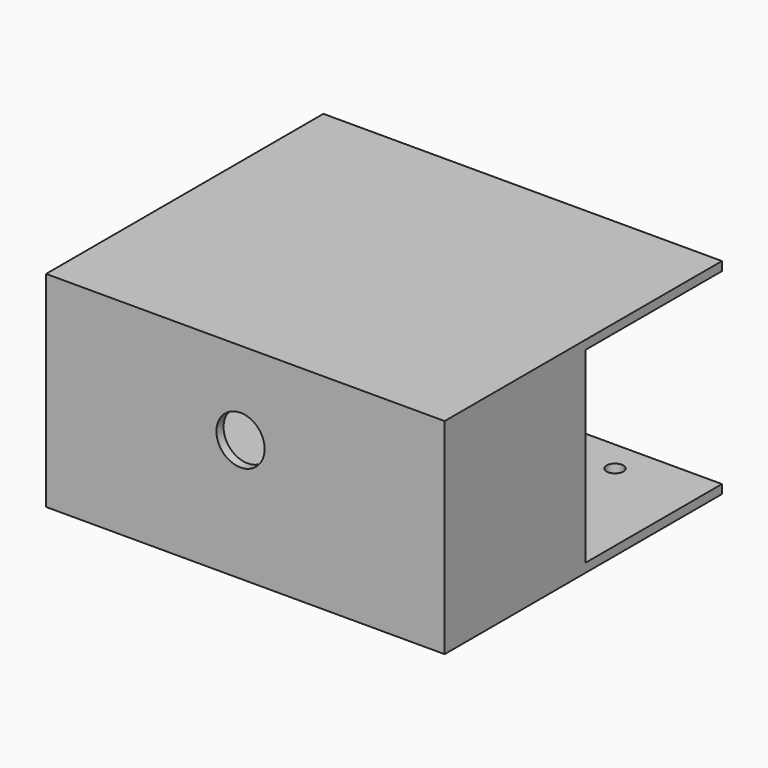
from build123d import *
from build123d import SkipClean  # not in build123d's __all__

# Parameters (mm, degrees)
F0_W             = 57.5
F0_H             = 50
F1_DEPTH         = 107.5
F2_W             = 55.8
F2_H             = 19
F3_DEPTH         = 42
F4_W             = 0.3
F4_H             = 19
F5_DEPTH         = 48.3
F6_T1_DEPTH      = 65.5
F6_T3_DEPTH      = 67.5
F6_T5_DEPTH      = 225
F6_T7_DEPTH      = 11.7
F6_T9_DEPTH      = 11.7
F6_T11_DEPTH     = 204
F8_W             = 87
F8_H             = 15.3
F9_DEPTH         = 14
F10_W            = 8.2
F10_H            = 14
F11_DEPTH        = 7.4
F12_R            = 2
F13_R            = 2.5
F14_DEPTH        = 4
F15_R            = 1
F19_D            = 3.3
F19_DEPTH        = 5
F19_TIP          = 0.9914200214
F19_ON_F18_D     = 3.3
F19_ON_F18_DEPTH = 5
F19_ON_F18_TIP   = 0.9914200214
F19_ON_F17_D     = 3.3
F19_ON_F17_DEPTH = 5
F19_ON_F17_TIP   = 0.9914200214
F20_W            = 264
F20_H            = 50
F20_R            = 1.5
F21_DEPTH        = 6
F22_W            = 122
F22_H            = 91
F22_R            = 2.25
F23_DEPTH        = 2.4
F24_W            = 91
F24_H            = 52.9
F24_R            = 1.75
F25_DEPTH        = 2.4
F26_R            = 2.25
F27_DEPTH        = 25
F28_W            = 91
F28_H            = 52.9
F29_DEPTH        = 3
F30_R            = 1.75
F31_DEPTH        = 25
F32_W            = 127.4
F32_H            = 91
F33_DEPTH        = 2.4
F34_W            = 127.4
F34_H            = 55.3
F34_R            = 6.5
F35_DEPTH        = 2.4
F36_W            = 21.5
F36_H            = 28.5
F37_DEPTH        = 25
F38_W            = 20
F38_H            = 100
F39_DEPTH        = 60
F43_W            = 2.4
F43_H            = 50.5
F44_DEPTH        = 45


# Not quite as in the source:
# - a fillet or chamfer that OpenCascade refuses, or shapes differently, is made with other operations: its cross-section is extruded or revolved along the edge and cut away or added


with BuildPart() as f1:
    # F0 (on Front) → F1 (new body, symmetric)
    with BuildSketch(Plane.XZ):
        with Locations((-28.75, 0)):
            Rectangle(F0_W, F0_H)
    extrude(amount=F1_DEPTH, both=True)

    # F2 (on face) → F3 (cut)
    with BuildSketch(Plane.XY.offset(25)):
        with Locations((-27.9, -98)):
            Rectangle(F2_W, F2_H)
    extrude(amount=-F3_DEPTH, mode=Mode.SUBTRACT)

    # F4 (on face) → F5 (cut)
    with BuildSketch(Plane.XY.offset(25)):
        Polygon((-55.8, 107.5), (-55.8, -88.5), (-55.5, -88.5), (-55.5, 105.5), (0, 105.5), (0, 105.8), (-55.5, 105.8), (-55.5, 107.5), align=None)
        with Locations((-55.65, -98)):
            Rectangle(F4_W, F4_H)
    extrude(amount=-F5_DEPTH, mode=Mode.SUBTRACT)

    # F6: fillet of radius 2 on 9 edges, made by hand

    # F6_s2 → F6_t1 (cut)
    with BuildSketch(Plane.YZ.offset(-60.5)):
        with BuildLine():
            ThreePointArc((-86.5, 25), (-87.9142135624, 24.4142135624), (-88.5, 23))
            Line((-88.5, 23), (-88.5, 25))
            Line((-88.5, 25), (-86.5, 25))
        make_face()
        with BuildLine():
            ThreePointArc((103.5, 25), (104.9142135624, 24.4142135624), (105.5, 23))
            Line((105.5, 23), (105.5, 25))
            Line((105.5, 25), (103.5, 25))
        make_face()
    extrude(amount=F6_T1_DEPTH, mode=Mode.SUBTRACT)

    # F6_s4 → F6_t3 (cut)
    with BuildSketch(Plane.YZ.offset(-62.5)):
        with BuildLine():
            ThreePointArc((-105.5, -25), (-106.9142135624, -24.4142135624), (-107.5, -23))
            Line((-107.5, -23), (-107.5, -25))
            Line((-107.5, -25), (-105.5, -25))
        make_face()
        with BuildLine():
            ThreePointArc((105.5, -25), (106.9142135624, -24.4142135624), (107.5, -23))
            Line((107.5, -23), (107.5, -25))
            Line((107.5, -25), (105.5, -25))
        make_face()
    extrude(amount=F6_T3_DEPTH, mode=Mode.SUBTRACT)

    # F6_s6 → F6_t5 (cut)
    with BuildSketch(Plane.XZ.offset(-112.5)):
        with BuildLine():
            ThreePointArc((-55.5, -25), (-56.9142135624, -24.4142135624), (-57.5, -23))
            Line((-57.5, -23), (-57.5, -25))
            Line((-57.5, -25), (-55.5, -25))
        make_face()
    extrude(amount=F6_T5_DEPTH, mode=Mode.SUBTRACT)

    # F6_s8 → F6_t7 (cut)
    with BuildSketch(Plane.YZ.offset(-62.5)):
        with BuildLine():
            ThreePointArc((-105.5, 25), (-106.9142135624, 24.4142135624), (-107.5, 23))
            Line((-107.5, 23), (-107.5, 25))
            Line((-107.5, 25), (-105.5, 25))
        make_face()
        with BuildLine():
            ThreePointArc((105.5, 25), (106.9142135624, 24.4142135624), (107.5, 23))
            Line((107.5, 23), (107.5, 25))
            Line((107.5, 25), (105.5, 25))
        make_face()
    extrude(amount=F6_T7_DEPTH, mode=Mode.SUBTRACT)

    # F6_s10 → F6_t9 (cut)
    with BuildSketch(Plane.XZ.offset(-112.5)):
        with BuildLine():
            ThreePointArc((-55.5, 23), (-54.9142135624, 24.4142135624), (-53.5, 25))
            Line((-53.5, 25), (-55.5, 25))
            Line((-55.5, 25), (-55.5, 23))
        make_face()
    extrude(amount=F6_T9_DEPTH, mode=Mode.SUBTRACT)

    # F6_s12 → F6_t11 (cut)
    with BuildSketch(Plane.XZ.offset(-110.5)):
        with BuildLine():
            ThreePointArc((-53.5, 25), (-54.9142135624, 24.4142135624), (-55.5, 23))
            Line((-55.5, 23), (-55.5, 25))
            Line((-55.5, 25), (-53.5, 25))
        make_face()
    with SkipClean():  # cleaning this boolean's faces spoils the solid; the shape is the same uncleaned
        extrude(amount=F6_T11_DEPTH, mode=Mode.SUBTRACT)

    # F7: F1 across plane


with BuildPart() as f1_1:
    add(f1.part, clean=False)
    add(f1.part.mirror(Plane.YZ), clean=False)

    # F19
    with Locations(Plane(origin=(-57.5, 0, 0), x_dir=(0, -1, 0), z_dir=(-1, 0, 0))):
        with Locations((-75, -13), (75, -13)):
            Hole(F19_D / 2, depth=F19_DEPTH)
            with Locations((0, 0, -(F19_DEPTH + F19_TIP / 2))):  # 118° drill point
                Cone(0, F19_D / 2, F19_TIP, mode=Mode.SUBTRACT)

    # F19 on F18
    with Locations(Plane(origin=(0, 0, -25), x_dir=(1, 0, 0), z_dir=(0, 0, -1))):
        with Locations((-25, -75), (-25, 75), (25, -75), (25, 75)):
            Hole(F19_ON_F18_D / 2, depth=F19_ON_F18_DEPTH)
            with Locations((0, 0, -(F19_ON_F18_DEPTH + F19_ON_F18_TIP / 2))):  # 118° drill point
                Cone(0, F19_ON_F18_D / 2, F19_ON_F18_TIP, mode=Mode.SUBTRACT)

    # F19 on F17
    with Locations(Plane.YZ.offset(57.5)):
        with Locations((-75, -13), (-75, 12), (75, 12), (75, -13)):
            Hole(F19_ON_F17_D / 2, depth=F19_ON_F17_DEPTH)
            with Locations((0, 0, -(F19_ON_F17_DEPTH + F19_ON_F17_TIP / 2))):  # 118° drill point
                Cone(0, F19_ON_F17_D / 2, F19_ON_F17_TIP, mode=Mode.SUBTRACT)


with BuildPart() as f9:
    # F8 (on face) → F9 (new body)
    with BuildSketch(Plane.XY.offset(-17)):
        with Locations((9.3, -96.15)):
            Rectangle(F8_W, F8_H)
    extrude(amount=F9_DEPTH)

    # F10 (on face) → F11 (cut)
    with BuildSketch(Plane.XY.offset(-3)):
        with Locations((-28.7, -96.8)):
            Rectangle(F10_W, F10_H)
        with Locations((-19.2, -96.8)):
            Rectangle(F10_W, F10_H)
        with Locations((-9.7, -96.8)):
            Rectangle(F10_W, F10_H)
        with Locations((-0.2, -96.8)):
            Rectangle(F10_W, F10_H)
        with Locations((9.3, -96.8)):
            Rectangle(F10_W, F10_H)
        with Locations((18.8, -96.8)):
            Rectangle(F10_W, F10_H)
        with Locations((28.3, -96.8)):
            Rectangle(F10_W, F10_H)
        with Locations((37.8, -96.8)):
            Rectangle(F10_W, F10_H)
        with Locations((47.3, -96.8)):
            Rectangle(F10_W, F10_H)
    extrude(amount=-F11_DEPTH, mode=Mode.SUBTRACT)

    # F12
    f12_edges = [f9.edges().sort_by_distance(p)[0] for p in [
        (-33.5, -103.8, -3),
        (-23.95, -103.8, -3),
        (-14.45, -103.8, -3),
        (-4.95, -103.8, -3),
        (4.55, -103.8, -3),
        (14.05, -103.8, -3),
        (23.55, -103.8, -3),
        (33.05, -103.8, -3),
        (42.55, -103.8, -3),
        (52.1, -103.8, -3),
    ]]
    fillet(f12_edges, radius=F12_R)

    # F13 (on face) → F14 (join)
    with BuildSketch(Plane.XY.offset(-10.4)):
        with Locations((-28.7, -96.8)):
            Circle(F13_R)
        with Locations((-19.2, -96.8)):
            Circle(F13_R)
        with Locations((-9.7, -96.8)):
            Circle(F13_R)
        with Locations((-0.2, -96.8)):
            Circle(F13_R)
        with Locations((9.3, -96.8)):
            Circle(F13_R)
        with Locations((18.8, -96.8)):
            Circle(F13_R)
        with Locations((28.3, -96.8)):
            Circle(F13_R)
        with Locations((37.8, -96.8)):
            Circle(F13_R)
        with Locations((47.3, -96.8)):
            Circle(F13_R)
    extrude(amount=F14_DEPTH)

    # F15
    f15_edges = [f9.edges().sort_by_distance(p)[0] for p in [
        (-31.2, -96.8, -6.4),
        (-21.7, -96.8, -6.4),
        (-12.2, -96.8, -6.4),
        (-2.7, -96.8, -6.4),
        (6.8, -96.8, -6.4),
        (16.3, -96.8, -6.4),
        (25.8, -96.8, -6.4),
        (35.3, -96.8, -6.4),
        (44.8, -96.8, -6.4),
    ]]
    fillet(f15_edges, radius=F15_R)


with BuildPart() as f21:
    # F20 (on face) → F21 (new body)
    with BuildSketch(Plane.YZ.offset(57.5)):
        with Locations((-24.5, 0)):
            Rectangle(F20_W, F20_H)
        with Locations((-75, -13)):
            Circle(F20_R, mode=Mode.SUBTRACT)
        with Locations((75, -13)):
            Circle(F20_R, mode=Mode.SUBTRACT)
        with Locations((-75, 12)):
            Circle(F20_R, mode=Mode.SUBTRACT)
        with Locations((75, 12)):
            Circle(F20_R, mode=Mode.SUBTRACT)
    extrude(amount=F21_DEPTH)


with BuildPart() as f23:
    # F22 (on face) → F23 (new body)
    with BuildSketch(Plane(origin=(0, 0, -25), x_dir=(1, 0, 0), z_dir=(0, 0, -1))):
        with Locations((3, 111.9773719933)):
            Rectangle(F22_W, F22_H)
        with Locations((-25, 75)):
            Circle(F22_R, mode=Mode.SUBTRACT)
        with Locations((25, 75)):
            Circle(F22_R, mode=Mode.SUBTRACT)
    extrude(amount=F23_DEPTH)

    # F24 (on face) → F25 (join)
    with BuildSketch(Plane(origin=(-58, 0, 0), x_dir=(0, -1, 0), z_dir=(-1, 0, 0))):
        with Locations((111.9773719933, -0.95)):
            Rectangle(F24_W, F24_H)
        with Locations((137.4773719933, -19.75)):
            Circle(F24_R, mode=Mode.SUBTRACT)
        with BuildLine():
            Line((127.4773719933, 9.25), (132.4773719933, 14.25))
            Line((132.4773719933, 14.25), (142.4773719933, 14.25))
            ThreePointArc((142.4773719933, 14.25), (146.0129058993, 12.7855339059), (147.4773719933, 9.25))
            Line((147.4773719933, 9.25), (147.4773719933, -8.75))
            ThreePointArc((147.4773719933, -8.75), (146.0129058993, -12.2855339059), (142.4773719933, -13.75))
            Line((142.4773719933, -13.75), (132.4773719933, -13.75))
            Line((132.4773719933, -13.75), (127.4773719933, -8.75))
            Line((127.4773719933, -8.75), (127.4773719933, 9.25))
        make_face(mode=Mode.SUBTRACT)
        with Locations((137.4773719933, 20.25)):
            Circle(F24_R, mode=Mode.SUBTRACT)
    extrude(amount=F25_DEPTH)

    # F26 (on face) → F27 (cut)
    with BuildSketch(Plane(origin=(-57.5, 0, 0), x_dir=(0, -1, 0), z_dir=(-1, 0, 0))):
        with Locations((75, -13)):
            Circle(F26_R)
    extrude(amount=F27_DEPTH, mode=Mode.SUBTRACT)

    # F28 (on face) → F29 (join)
    with BuildSketch(Plane.YZ.offset(64)):
        with Locations((-111.9773719933, -0.95)):
            Rectangle(F28_W, F28_H)
    extrude(amount=F29_DEPTH)

    # F30 (on face) → F31 (cut)
    with BuildSketch(Plane.YZ.offset(63.5)):
        with Locations((-75, 12)):
            Circle(F30_R)
        with Locations((-75, -13)):
            Circle(F30_R)
    extrude(amount=F31_DEPTH, mode=Mode.SUBTRACT)

    # F32 (on face) → F33 (join)
    with BuildSketch(Plane.XY.offset(25.5)):
        with Locations((3.3, -111.9773719933)):
            Rectangle(F32_W, F32_H)
    extrude(amount=F33_DEPTH)

    # F34 (on face) → F35 (join)
    with BuildSketch(Plane.XZ.offset(157.4773719933)):
        with Locations((3.3, 0.25)):
            Rectangle(F34_W, F34_H)
        with Locations((-8, 5.5)):
            Circle(F34_R, mode=Mode.SUBTRACT)
    extrude(amount=F35_DEPTH)

    # F36 (on face) → F37 (cut)
    with BuildSketch(Plane(origin=(0, 0, -27.4), x_dir=(1, 0, 0), z_dir=(0, 0, -1))):
        with Locations((16.25, 133.2273719933)):
            Rectangle(F36_W, F36_H)
    extrude(amount=-F37_DEPTH, mode=Mode.SUBTRACT)


with BuildPart() as f39_tool:
    # F38 (on face) → F39 (new body)
    with BuildSketch(Plane.XY.offset(27.9)):
        with Locations((57, -109.8773719933)):
            Rectangle(F38_W, F38_H)
    extrude(amount=-F39_DEPTH)


with BuildPart() as f1_2:
    add(f1_1.part, clean=False)

    # F39: cut by f39_tool
    add(f39_tool.part, mode=Mode.SUBTRACT)


with BuildPart() as f9_1:
    add(f9.part, clean=False)

    # F39: cut by f39_tool
    add(f39_tool.part, mode=Mode.SUBTRACT)


with BuildPart() as f21_1:
    add(f21.part, clean=False)

    # F39: cut by f39_tool
    add(f39_tool.part, mode=Mode.SUBTRACT)


with BuildPart() as f23_1:
    add(f23.part, clean=False)

    # F39: cut by f39_tool
    add(f39_tool.part, mode=Mode.SUBTRACT)

    # F43 (on face) → F44 (join)
    with BuildSketch(Plane(origin=(0, -157.4773719933, 0), x_dir=(-1, 0, 0), z_dir=(0, 1, 0))):
        with Locations((-45.8, 0.25)):
            Rectangle(F43_W, F43_H)
    extrude(amount=F44_DEPTH)


solid = f23_1.part
